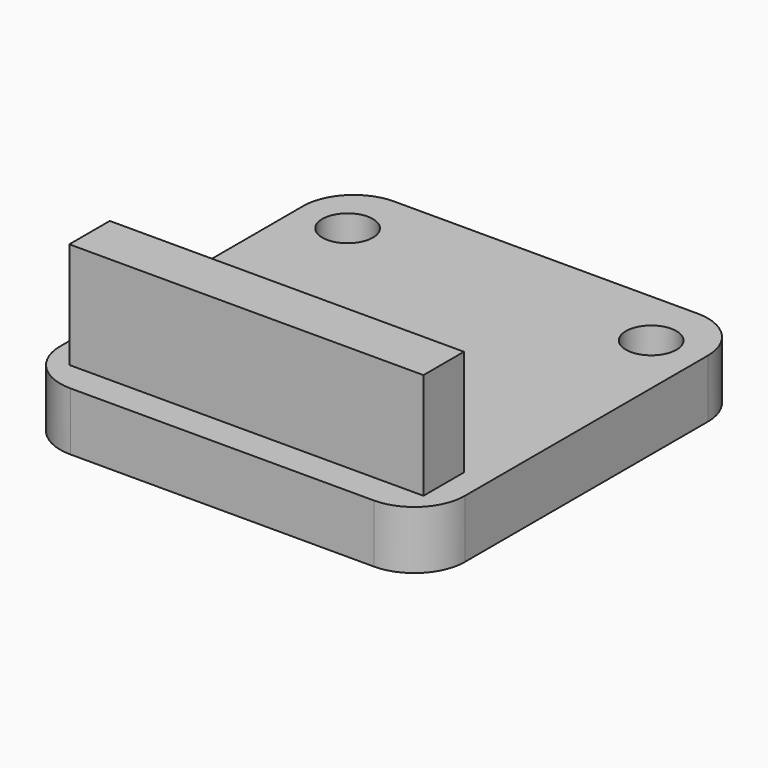
from build123d import *

# Parameters (mm, degrees)
F0_W     = 20.32
F0_H     = 20.32
F1_DEPTH = 2.921
F3_D     = 2.54
F5_R     = 2.54
F4_W     = 17.78
F4_H     = 2.54
F6_DEPTH = 5.334
F8_D     = 1.27


# Not quite as in the source:
# - a pattern or mirror of a feature is missing from the dataset's text; its kind, count and spacing are read off the source's solid


with BuildPart() as f1:
    # F0 (on Top) → F1 (new body)
    with BuildSketch(Plane.XY):
        Rectangle(F0_W, F0_H)
    extrude(amount=F1_DEPTH)

    # F3 (through all)
    with Locations(Plane.XY.offset(2.921)):
        with Locations((-7.62, 7.2416714393)):
            f3 = Hole(F3_D / 2)

    # F3_copies: F3 across plane
    add(f3.mirror(Plane(origin=(0, 0, 0), x_dir=(0, 0, 1), z_dir=(1, 0, 0))), mode=Mode.SUBTRACT)

    # F5
    f5_edges = [f1.edges().sort_by_distance(p)[0] for p in [
        (-10.16, 10.16, 1.4605),
        (10.16, 10.16, 1.4605),
        (-10.16, -10.16, 1.4605),
        (10.16, -10.16, 1.4605),
    ]]
    fillet(f5_edges, radius=F5_R)

    # F4 (on face) → F6 (join)
    with BuildSketch(Plane.XY.offset(2.921)):
        with Locations((0, -7.366)):
            Rectangle(F4_W, F4_H)
    extrude(amount=F6_DEPTH)

    # F8 (through all)
    with Locations(Plane.XY.offset(2.921)):
        with Locations((0, 0)):
            Hole(F8_D / 2)


solid = f1.part
